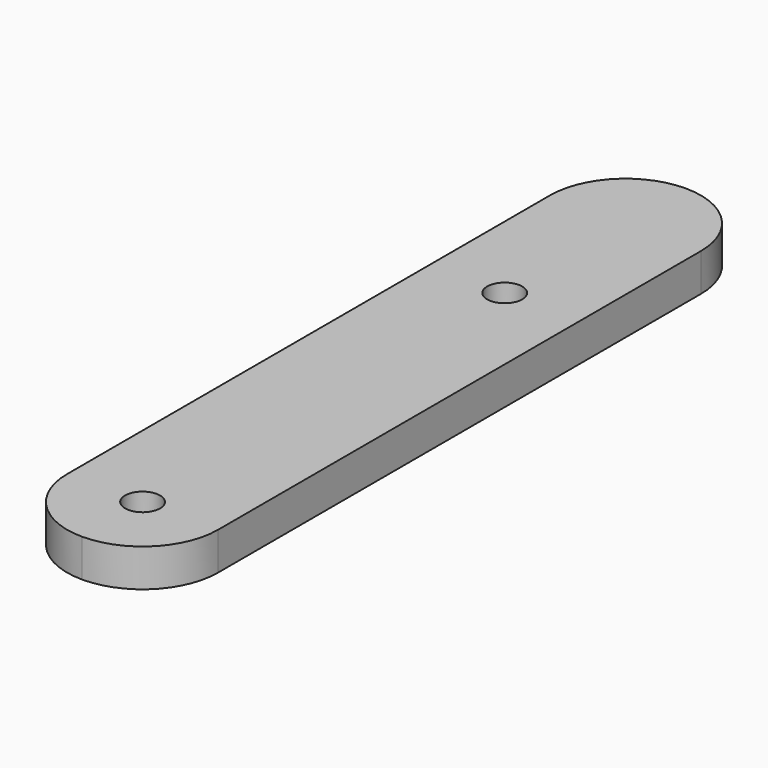
from build123d import *

# Parameters (mm, degrees)
F0_R     = 1.4732
F1_DEPTH = 3.175


# Not quite as in the source:
# - a length typed as a fraction of an inch, garbled in the dataset ("3 / 203.2 mm" for 3/8 in), is restored


with BuildPart() as f1:
    # F0 (on Top) → F1 (new body)
    with BuildSketch(Plane.XY):
        with BuildLine():
            Line((6.35, -19.05), (6.35, 25.4))
            Line((6.35, 25.4), (6.35, 31.75))
            ThreePointArc((6.35, 31.75), (4.4901280605, 36.2401280605), (0, 38.1))
            ThreePointArc((0, 38.1), (-4.4901280605, 36.2401280605), (-6.35, 31.75))
            Line((-6.35, 31.75), (-6.35, 25.4))
            Line((-6.35, 25.4), (-6.35, -19.05))
            ThreePointArc((-6.35, -19.05), (-4.4901280605, -23.5401280605), (0, -25.4))
            ThreePointArc((0, -25.4), (4.4901280605, -23.5401280605), (6.35, -19.05))
        make_face()
        with Locations((0, -19.05)):
            Circle(F0_R, mode=Mode.SUBTRACT)
        with Locations((0, 19.05)):
            Circle(F0_R, mode=Mode.SUBTRACT)
    extrude(amount=F1_DEPTH)


solid = f1.part
